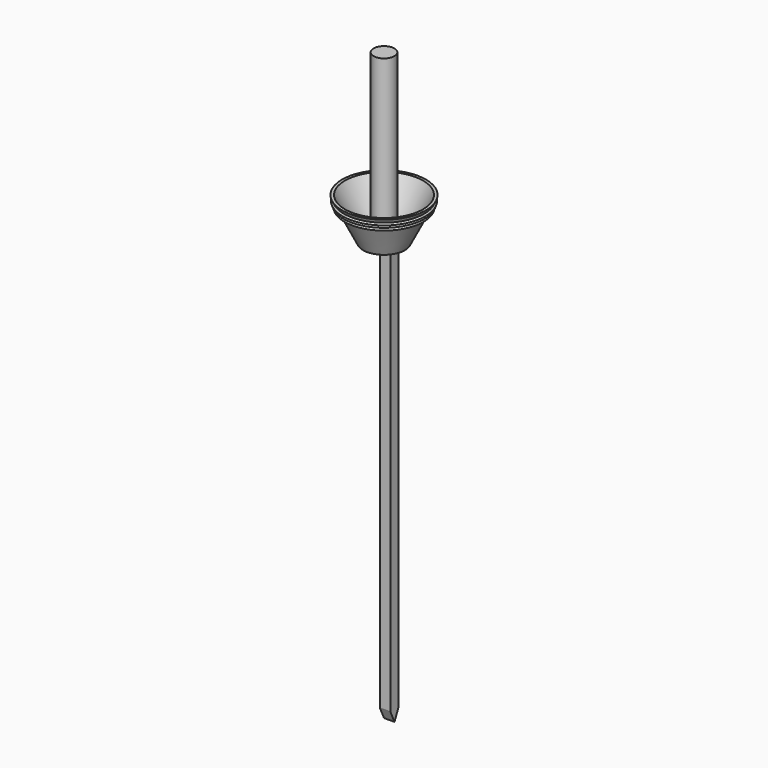
from build123d import *

# Parameters (mm, degrees)
F2_W     = 12.7
F2_H     = 508
F3_DEPTH = 6.35
F5_DEPTH = 25.399999693
F6_W     = 12.7
F6_H     = 203.2


with BuildPart() as f1:
    # F0 (on Right) → F1 (revolve)
    with BuildSketch(Plane.YZ):
        Polygon((0, 3.0734), (0, 0), (25.4, 0), (44.7754811435, 38.750962287), (48.59950418, 46.3990083599), (50.8, 50.8), (47.363834339, 50.8), (23.500534339, 3.0734), align=None)
        Polygon((48.59950418, 46.3990083599), (44.7754811435, 38.750962287), (47.9032658041, 37.5654287636), (46.203892678, 41.5475443006), (49.1207279265, 41.167087853), (47.5989021361, 44.1600158811), (50.2621009946, 44.362924993), align=None)
    revolve(axis=Axis((0, 0, 25.4), (0, 0, -1)))

    # F2 (on Front) → F3 (join, symmetric)
    with BuildSketch(Plane.XZ):
        with Locations((6.35, -254)):
            Rectangle(F2_W, F2_H)
    extrude(amount=F3_DEPTH, both=True)

    # F4 (on face) → F5 (cut)
    with BuildSketch(Plane(origin=(0, 0, 0), x_dir=(0, -1, 0), z_dir=(-1, 0, 0))):
        Polygon((6.35, -494.3823810548), (0, -508), (6.35, -508), align=None)
        Polygon((-6.35, -508), (0, -508), (-6.35, -494.3823810548), align=None)
    extrude(amount=-F5_DEPTH, mode=Mode.SUBTRACT)

    # F6 (on Front) → F8 (revolve)
    with BuildSketch(Plane.XZ):
        with Locations((6.35, 101.6)):
            Rectangle(F6_W, F6_H)
    revolve(axis=Axis((0, 0, 101.6), (0, 0, 1)))


with BuildPart() as f7:
    # F6 (on Front) → F7 (revolve)
    with BuildSketch(Plane.XZ):
        with Locations((6.35, 101.6)):
            Rectangle(F6_W, F6_H)
    revolve(axis=Axis((0, 0, 101.6), (0, 0, 1)))


solid = Compound([f1.part, f7.part])
